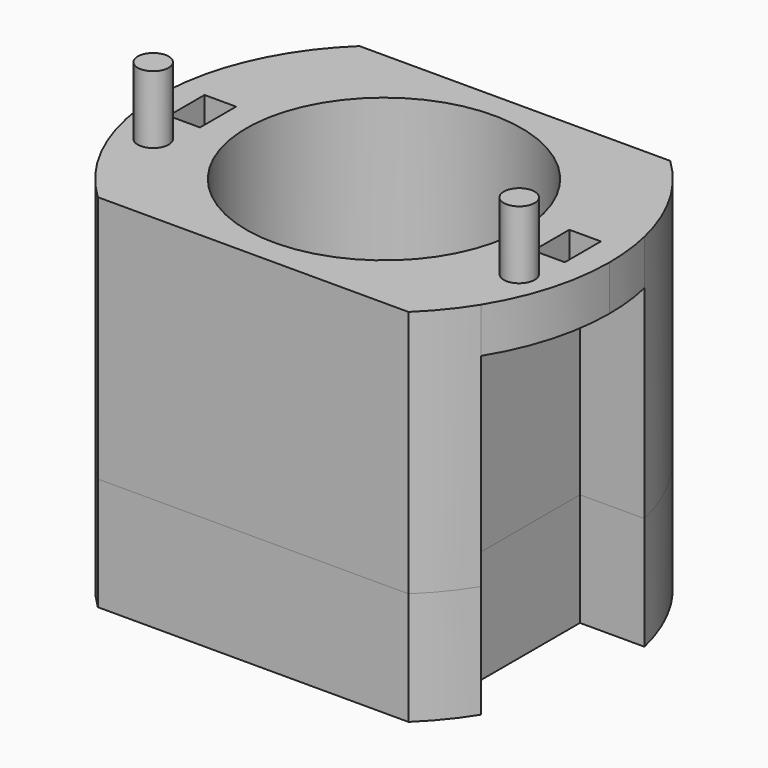
from build123d import *

# Parameters (mm, degrees)
F0_R     = 30.5
F1_DEPTH = 45
F0_R_2   = 3.425
F0_W     = 7
F0_H     = 10
F2_DEPTH = 10
F3_DEPTH = 25
F5_DEPTH = 25


# Not quite as in the source:
# - a feature names something its author has since deleted; it is built from what else it names


with BuildPart() as f1:
    # F0 (on Top) → F1 (new body)
    with BuildSketch(Plane.XY):
        Polygon((34.4299112098, 11.2571539711), (34.4299112098, 36.2571539711), (-34.4299112098, 36.2571539711), (-34.4299112098, 11.2571539711), (-34.4299112098, -26.2571539711), (-34.4299112098, -36.2571539711), (34.4299112098, -36.2571539711), (34.4299112098, -26.2571539711), align=None)
        Circle(F0_R, mode=Mode.SUBTRACT)
        with BuildLine():
            Line((-34.4299112098, 11.2571539711), (-34.4299112098, 36.2571539711))
            ThreePointArc((-34.4299112098, 36.2571539711), (-43.4116633148, 24.8078110329), (-48.7162856186, 11.2571539711))
            Line((-48.7162856186, 11.2571539711), (-34.4299112098, 11.2571539711))
        make_face()
        with BuildLine():
            Line((34.4299112098, 11.2571539711), (48.7162856186, 11.2571539711))
            ThreePointArc((48.7162856186, 11.2571539711), (43.4116633148, 24.8078110329), (34.4299112098, 36.2571539711))
            Line((34.4299112098, 36.2571539711), (34.4299112098, 11.2571539711))
        make_face()
        with BuildLine():
            ThreePointArc((34.4299112098, -36.2571539711), (38.8137028995, -31.5197789844), (42.5506975893, -26.2571539711))
            Line((42.5506975893, -26.2571539711), (34.4299112098, -26.2571539711))
            Line((34.4299112098, -26.2571539711), (34.4299112098, -36.2571539711))
        make_face()
        with BuildLine():
            ThreePointArc((-42.5506975893, -26.2571539711), (-38.8137028995, -31.5197789844), (-34.4299112098, -36.2571539711))
            Line((-34.4299112098, -36.2571539711), (-34.4299112098, -26.2571539711))
            Line((-34.4299112098, -26.2571539711), (-42.5506975893, -26.2571539711))
        make_face()
    extrude(amount=-F1_DEPTH)

    # F0 (on Top) → F2 (join)
    with BuildSketch(Plane.XY):
        Polygon((34.4299112098, 11.2571539711), (34.4299112098, 36.2571539711), (-34.4299112098, 36.2571539711), (-34.4299112098, 11.2571539711), (-34.4299112098, -26.2571539711), (-34.4299112098, -36.2571539711), (34.4299112098, -36.2571539711), (34.4299112098, -26.2571539711), align=None)
        Circle(F0_R, mode=Mode.SUBTRACT)
        with BuildLine():
            Line((-34.4299112098, 11.2571539711), (-48.7162856186, 11.2571539711))
            ThreePointArc((-48.7162856186, 11.2571539711), (-49.3380824624, -8.1088605202), (-42.5506975893, -26.2571539711))
            Line((-42.5506975893, -26.2571539711), (-34.4299112098, -26.2571539711))
            Line((-34.4299112098, -26.2571539711), (-34.4299112098, 11.2571539711))
        make_face()
        with Locations((-40.5626991825, -13.233267504)):
            Circle(F0_R_2, mode=Mode.SUBTRACT)
        with Locations((-40.4299112098, 0.191732496)):
            Rectangle(F0_W, F0_H, mode=Mode.SUBTRACT)
        with BuildLine():
            ThreePointArc((42.5506975893, -26.2571539711), (48.1016365598, -13.6467051066), (50, 0))
            ThreePointArc((50, 0), (49.6780347887, 5.6650560046), (48.7162856186, 11.2571539711))
            Line((48.7162856186, 11.2571539711), (34.4299112098, 11.2571539711))
            Line((34.4299112098, 11.2571539711), (34.4299112098, -26.2571539711))
            Line((34.4299112098, -26.2571539711), (42.5506975893, -26.2571539711))
        make_face()
        with Locations((40.5626991825, -13.233267504)):
            Circle(F0_R_2, mode=Mode.SUBTRACT)
        with Locations((40.4299112098, 0.191732496)):
            Rectangle(F0_W, F0_H, mode=Mode.SUBTRACT)
        with BuildLine():
            Line((34.4299112098, 11.2571539711), (48.7162856186, 11.2571539711))
            ThreePointArc((48.7162856186, 11.2571539711), (43.4116633148, 24.8078110329), (34.4299112098, 36.2571539711))
            Line((34.4299112098, 36.2571539711), (34.4299112098, 11.2571539711))
        make_face()
        with BuildLine():
            Line((-34.4299112098, 11.2571539711), (-34.4299112098, 36.2571539711))
            ThreePointArc((-34.4299112098, 36.2571539711), (-43.4116633148, 24.8078110329), (-48.7162856186, 11.2571539711))
            Line((-48.7162856186, 11.2571539711), (-34.4299112098, 11.2571539711))
        make_face()
        with BuildLine():
            ThreePointArc((34.4299112098, -36.2571539711), (38.8137028995, -31.5197789844), (42.5506975893, -26.2571539711))
            Line((42.5506975893, -26.2571539711), (34.4299112098, -26.2571539711))
            Line((34.4299112098, -26.2571539711), (34.4299112098, -36.2571539711))
        make_face()
        with BuildLine():
            ThreePointArc((-42.5506975893, -26.2571539711), (-38.8137028995, -31.5197789844), (-34.4299112098, -36.2571539711))
            Line((-34.4299112098, -36.2571539711), (-34.4299112098, -26.2571539711))
            Line((-34.4299112098, -26.2571539711), (-42.5506975893, -26.2571539711))
        make_face()
        with Locations((-40.5626991825, -13.233267504)):
            Circle(F0_R_2)
        with Locations((40.5626991825, -13.233267504)):
            Circle(F0_R_2)
    extrude(amount=F2_DEPTH)

    # F0 (on Top) → F3 (join)
    with BuildSketch(Plane.XY):
        with Locations((-40.5626991825, -13.233267504)):
            Circle(F0_R_2)
        with Locations((40.5626991825, -13.233267504)):
            Circle(F0_R_2)
    extrude(amount=F3_DEPTH)

    # F4 (on face) → F5 (join)
    with BuildSketch(Plane(origin=(0, 0, -45), x_dir=(1, 0, 0), z_dir=(0, 0, -1))):
        Polygon((-34.4299112098, -36.2571539711), (34.4299112098, -36.2571539711), (34.4299112098, -11.2571539711), (34.4299112098, 26.2571539711), (34.4299112098, 36.2571539711), (-34.4299112098, 36.2571539711), (-34.4299112098, 26.2571539711), (-34.4299112098, -11.2571539711), align=None)
        Polygon((0, 30.5), (30.5, 30.5), (30.5, 0), (30.5, -30.5), (-3.98e-08, -30.5), (-30.5, -30.5), (-30.5, 4.66e-08), (-30.5, 30.5), align=None, mode=Mode.SUBTRACT)
        with BuildLine():
            Line((34.4299112098, -11.2571539711), (34.4299112098, -36.2571539711))
            ThreePointArc((34.4299112098, -36.2571539711), (43.4116633148, -24.8078110329), (48.7162856186, -11.2571539711))
            Line((48.7162856186, -11.2571539711), (34.4299112098, -11.2571539711))
        make_face()
        with BuildLine():
            ThreePointArc((-48.7162856186, -11.2571539711), (-43.4116633148, -24.8078110329), (-34.4299112098, -36.2571539711))
            Line((-34.4299112098, -36.2571539711), (-34.4299112098, -11.2571539711))
            Line((-34.4299112098, -11.2571539711), (-48.7162856186, -11.2571539711))
        make_face()
        with BuildLine():
            Line((-42.5506975893, 26.2571539711), (-34.4299112098, 26.2571539711))
            Line((-34.4299112098, 26.2571539711), (-34.4299112098, 36.2571539711))
            ThreePointArc((-34.4299112098, 36.2571539711), (-38.8137028995, 31.5197789844), (-42.5506975893, 26.2571539711))
        make_face()
        with BuildLine():
            Line((34.4299112098, 36.2571539711), (34.4299112098, 26.2571539711))
            Line((34.4299112098, 26.2571539711), (42.5506975893, 26.2571539711))
            ThreePointArc((42.5506975893, 26.2571539711), (38.8137028995, 31.5197789844), (34.4299112098, 36.2571539711))
        make_face()
    extrude(amount=F5_DEPTH)


solid = f1.part
